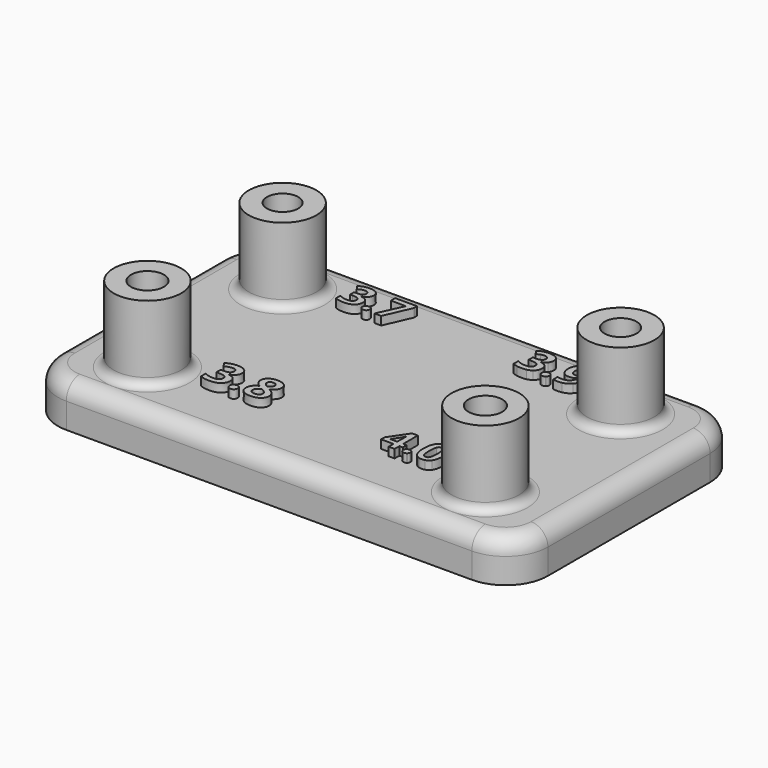
from build123d import *

# Parameters (mm, degrees)
F0_R           = 4
F0_R_2         = 1.85
F1_DEPTH       = 12
F0_R_3         = 1.95
F0_R_4         = 2
F0_R_5         = 1.9
F2_W           = 58
F2_H           = 34
F3_DEPTH       = 5
F5_R           = 5
F6_TEXT_SIZE   = 5.0406240237
F6_TEXT_SIZE_2 = 5.4685932377
F7_DEPTH       = 6
F9_R           = 2
F10_R          = 0.99999


# Not quite as in the source:
# - a fillet or chamfer is up to 0.001 mm smaller than in the source, because OpenCascade refuses the exact size
# - Text() gives the source's letters only with a copy of the font that has no kerning and outlines rounded to 1/6400 em; it was checked with that copy


with BuildPart() as f1:
    # F0 (on Top) → F1 (new body)
    with BuildSketch(Plane.XY):
        with Locations((-20, 10)):
            Circle(F0_R)
        with Locations((-20, 10)):
            Circle(F0_R_2, mode=Mode.SUBTRACT)
    extrude(amount=F1_DEPTH)


with BuildPart() as f1b:
    # F0 (on Top) → F1, piece 2 (new body)
    with BuildSketch(Plane.XY):
        with Locations((-20, -10)):
            Circle(F0_R)
        with Locations((-20, -10)):
            Circle(F0_R_3, mode=Mode.SUBTRACT)
    extrude(amount=F1_DEPTH)


with BuildPart() as f1c:
    # F0 (on Top) → F1, piece 3 (new body)
    with BuildSketch(Plane.XY):
        with Locations((20, -10)):
            Circle(F0_R)
        with Locations((20, -10)):
            Circle(F0_R_4, mode=Mode.SUBTRACT)
    extrude(amount=F1_DEPTH)


with BuildPart() as f1d:
    # F0 (on Top) → F1, piece 4 (new body)
    with BuildSketch(Plane.XY):
        with Locations((20, 10)):
            Circle(F0_R)
        with Locations((20, 10)):
            Circle(F0_R_5, mode=Mode.SUBTRACT)
    extrude(amount=F1_DEPTH)


with BuildPart() as f3:
    # F2 (on Top) → F3 (new body)
    with BuildSketch(Plane.XY):
        Rectangle(F2_W, F2_H)
    extrude(amount=F3_DEPTH)

    # F5
    f5_edges = [f3.edges().sort_by_distance(p)[0] for p in [
        (29, -17, 2.5),
        (-29, -17, 2.5),
        (-29, 17, 2.5),
        (29, 17, 2.5),
    ]]
    fillet(f5_edges, radius=F5_R)

    # F6 (on Top) → F7 (join)
    with BuildSketch(Plane.XY):
        with BuildLine():
            add(Edge.make_bspline(
                [(8.8647170825, 10), (8.6159599899, 9.9472579578), (8.308504951, 9.9472579578)],
                knots=[0.5859606644, 0.5859606644, 0.5859606644, 1, 1, 1], degree=2))
            Line((8.8647170825, 10), (7.7154605589, 10))
            add(Edge.make_bspline(
                [(8.308504951, 9.9472579578), (7.9939394248, 9.9472579578), (7.7154605589, 10)],
                knots=[0, 0, 0, 0.5050353738, 0.5050353738, 0.5050353738], degree=2))
        make_face()
        with BuildLine():
            Line((7.7154605589, 10), (8.8647170825, 10))
            add(Edge.make_bspline(
                [(9.4512491981, 10.2549198705), (9.2167654477, 10.0746420917), (8.8647170825, 10)],
                knots=[0, 0, 0, 0.5859606644, 0.5859606644, 0.5859606644], degree=2))
            add(Edge.make_bspline(
                [(9.8514189783, 11.1142802878), (9.8514189783, 10.5625817832), (9.4512491981, 10.2549198705)],
                knots=[0, 0, 0, 1, 1, 1], degree=2))
            add(Edge.make_bspline(
                [(9.6136612009, 11.7174650717), (9.8514189783, 11.4935206862), (9.8514189783, 11.1142802878)],
                knots=[0, 0, 0, 1, 1, 1], degree=2))
            add(Edge.make_bspline(
                [(8.9121083225, 11.9991745509), (9.3759034235, 11.9414094571), (9.6136612009, 11.7174650717)],
                knots=[0, 0, 0, 1, 1, 1], degree=2))
            Line((8.9121083225, 11.9991745509), (8.9121083225, 12.0142437058))
            add(Edge.make_bspline(
                [(9.5219905086, 12.3599970933), (9.3047435254, 12.1088445116), (8.9121083225, 12.0142437058)],
                knots=[0, 0, 0, 1, 1, 1], degree=2))
            add(Edge.make_bspline(
                [(9.7392374918, 12.9694606918), (9.7392374918, 12.6111496751), (9.5219905086, 12.3599970933)],
                knots=[0, 0, 0, 1, 1, 1], degree=2))
            add(Edge.make_bspline(
                [(9.3951584548, 13.6387823222), (9.7392374918, 13.3980944313), (9.7392374918, 12.9694606918)],
                knots=[0, 0, 0, 1, 1, 1], degree=2))
            add(Edge.make_bspline(
                [(8.4575221495, 13.879470213), (9.0510794178, 13.879470213), (9.3951584548, 13.6387823222)],
                knots=[0, 0, 0, 1, 1, 1], degree=2))
            add(Edge.make_bspline(
                [(7.2092938181, 13.5027413404), (7.7325283635, 13.879470213), (8.4575221495, 13.879470213)],
                knots=[0, 0, 0, 1, 1, 1], degree=2))
            Line((7.2092938181, 13.5027413404), (7.583511165, 12.9460197841))
            add(Edge.make_bspline(
                [(8.0163307809, 13.1628481797), (7.8212689424, 13.1000600343), (7.583511165, 12.9460197841)],
                knots=[0, 0, 0, 1, 1, 1], degree=2))
            add(Edge.make_bspline(
                [(8.3997570557, 13.2256363252), (8.2113926194, 13.2256363252), (8.0163307809, 13.1628481797)],
                knots=[0, 0, 0, 1, 1, 1], degree=2))
            add(Edge.make_bspline(
                [(8.9439209829, 12.7911423587), (8.9439209829, 13.2256363252), (8.3997570557, 13.2256363252)],
                knots=[0, 0, 0, 1, 1, 1], degree=2))
            add(Edge.make_bspline(
                [(8.7383944535, 12.392646929), (8.9439209829, 12.5090142919), (8.9439209829, 12.7911423587)],
                knots=[0, 0, 0, 1, 1, 1], degree=2))
            add(Edge.make_bspline(
                [(8.0883278543, 12.2762795661), (8.5328679241, 12.2762795661), (8.7383944535, 12.392646929)],
                knots=[0, 0, 0, 1, 1, 1], degree=2))
            Line((8.0883278543, 12.2762795661), (7.7928049831, 12.2762795661))
            Line((7.7928049831, 12.2762795661), (7.7928049831, 11.6559326891))
            Line((7.7928049831, 11.6559326891), (8.0833048027, 11.6559326891))
            add(Edge.make_bspline(
                [(8.7844390935, 11.543332615), (8.5646805844, 11.6559326891), (8.0833048027, 11.6559326891)],
                knots=[0, 0, 0, 1, 1, 1], degree=2))
            add(Edge.make_bspline(
                [(9.0041976025, 11.1619992783), (9.0041976025, 11.4307325408), (8.7844390935, 11.543332615)],
                knots=[0, 0, 0, 1, 1, 1], degree=2))
            add(Edge.make_bspline(
                [(8.8133216404, 10.7245751984), (9.0041976025, 10.8606161802), (9.0041976025, 11.1619992783)],
                knots=[0, 0, 0, 1, 1, 1], degree=2))
            add(Edge.make_bspline(
                [(8.2214387227, 10.5885342166), (8.6224456782, 10.5885342166), (8.8133216404, 10.7245751984)],
                knots=[0, 0, 0, 1, 1, 1], degree=2))
            add(Edge.make_bspline(
                [(7.6931811257, 10.6592755271), (7.9602400376, 10.5885342166), (8.2214387227, 10.5885342166)],
                knots=[0, 0, 0, 1, 1, 1], degree=2))
            add(Edge.make_bspline(
                [(7.2042707665, 10.8421983242), (7.4261222137, 10.7300168377), (7.6931811257, 10.6592755271)],
                knots=[0, 0, 0, 1, 1, 1], degree=2))
            Line((7.2042707665, 10.8421983242), (7.2042707665, 10.1540402502))
            add(Edge.make_bspline(
                [(7.7154605589, 10), (7.4425347504, 10.0516903301), (7.2042707665, 10.1540402502)],
                knots=[0.5050353738, 0.5050353738, 0.5050353738, 1, 1, 1], degree=2))
        make_face()
        with BuildLine():
            add(Edge.make_bspline(
                [(11.0990122142, 10), (10.9898897297, 9.9296772771), (10.8250538203, 9.9296772771)],
                knots=[0.2308775808, 0.2308775808, 0.2308775808, 1, 1, 1], degree=2))
            Line((11.0990122142, 10), (10.5431894654, 10))
            add(Edge.make_bspline(
                [(10.8250538203, 9.9296772771), (10.6538929904, 9.9296772771), (10.5431894654, 10)],
                knots=[0, 0, 0, 0.7773779948, 0.7773779948, 0.7773779948], degree=2))
        make_face()
        with BuildLine():
            Line((10.5431894654, 10), (11.0990122142, 10))
            add(Edge.make_bspline(
                [(11.1595053417, 10.0485561658), (11.131768944, 10.0211096956), (11.0990122142, 10)],
                knots=[0, 0, 0, 0.2308775808, 0.2308775808, 0.2308775808], degree=2))
            add(Edge.make_bspline(
                [(11.2796399933, 10.3742173468), (11.2796399933, 10.1674350545), (11.1595053417, 10.0485561658)],
                knots=[0, 0, 0, 1, 1, 1], degree=2))
            add(Edge.make_bspline(
                [(11.1607611046, 10.7036458166), (11.2796399933, 10.5885342166), (11.2796399933, 10.3742173468)],
                knots=[0, 0, 0, 1, 1, 1], degree=2))
            add(Edge.make_bspline(
                [(10.8250538203, 10.8187574166), (11.0418822159, 10.8187574166), (11.1607611046, 10.7036458166)],
                knots=[0, 0, 0, 1, 1, 1], degree=2))
            add(Edge.make_bspline(
                [(10.4822305462, 10.7061573424), (10.599853672, 10.8187574166), (10.8250538203, 10.8187574166)],
                knots=[0, 0, 0, 1, 1, 1], degree=2))
            add(Edge.make_bspline(
                [(10.3646074204, 10.3742173468), (10.3646074204, 10.5935572682), (10.4822305462, 10.7061573424)],
                knots=[0, 0, 0, 1, 1, 1], degree=2))
            add(Edge.make_bspline(
                [(10.484742072, 10.04604464), (10.3646074204, 10.1624120029), (10.3646074204, 10.3742173468)],
                knots=[0, 0, 0, 1, 1, 1], degree=2))
            add(Edge.make_bspline(
                [(10.5431894654, 10), (10.5114866891, 10.0201387043), (10.484742072, 10.04604464)],
                knots=[0.7773779948, 0.7773779948, 0.7773779948, 1, 1, 1], degree=2))
        make_face()
        with BuildLine():
            add(Edge.make_bspline(
                [(13.0887324097, 10), (12.838141706, 9.9472579578), (12.5412631291, 9.9472579578)],
                knots=[0.6924376574, 0.6924376574, 0.6924376574, 1, 1, 1], degree=2))
            Line((13.0887324097, 10), (12.0255631612, 10))
            Line((12.0255631612, 10), (12.0255631612, 9.9840936698))
            add(Edge.make_bspline(
                [(12.5412631291, 9.9472579578), (12.2005327931, 9.9472579578), (12.0255631612, 9.9840936698)],
                knots=[0, 0, 0, 1, 1, 1], degree=2))
        make_face()
        with BuildLine():
            Line((12.0255631612, 10), (13.0887324097, 10))
            add(Edge.make_bspline(
                [(13.9824603608, 10.5048166894), (13.6529056381, 10.1187420274), (13.0887324097, 10)],
                knots=[0, 0, 0, 0.6924376574, 0.6924376574, 0.6924376574], degree=2))
            add(Edge.make_bspline(
                [(14.4583945032, 12.1925620388), (14.4583945032, 11.0623754209), (13.9824603608, 10.5048166894)],
                knots=[0, 0, 0, 1, 1, 1], degree=2))
            add(Edge.make_bspline(
                [(14.2884479229, 13.0937812197), (14.4583945032, 12.7157965842), (14.4583945032, 12.1925620388)],
                knots=[0, 0, 0, 1, 1, 1], degree=2))
            add(Edge.make_bspline(
                [(13.8007933266, 13.6705949825), (14.1185013426, 13.4717658553), (14.2884479229, 13.0937812197)],
                knots=[0, 0, 0, 1, 1, 1], degree=2))
            add(Edge.make_bspline(
                [(13.0586374475, 13.8694241098), (13.4830853107, 13.8694241098), (13.8007933266, 13.6705949825)],
                knots=[0, 0, 0, 1, 1, 1], degree=2))
            add(Edge.make_bspline(
                [(12.1080249255, 13.512368856), (12.4575456018, 13.8694241098), (13.0586374475, 13.8694241098)],
                knots=[0, 0, 0, 1, 1, 1], degree=2))
            add(Edge.make_bspline(
                [(11.7585042492, 12.5399897769), (11.7585042492, 13.1553136023), (12.1080249255, 13.512368856)],
                knots=[0, 0, 0, 1, 1, 1], degree=2))
            add(Edge.make_bspline(
                [(12.046492543, 11.6496538746), (11.7585042492, 11.9698734163), (11.7585042492, 12.5399897769)],
                knots=[0, 0, 0, 1, 1, 1], degree=2))
            add(Edge.make_bspline(
                [(12.8342744745, 11.3294343328), (12.3344808368, 11.3294343328), (12.046492543, 11.6496538746)],
                knots=[0, 0, 0, 1, 1, 1], degree=2))
            add(Edge.make_bspline(
                [(13.3311379987, 11.4286396026), (13.1323088715, 11.3294343328), (12.8342744745, 11.3294343328)],
                knots=[0, 0, 0, 1, 1, 1], degree=2))
            add(Edge.make_bspline(
                [(13.6814958503, 11.7739744026), (13.529967126, 11.5278448724), (13.3311379987, 11.4286396026)],
                knots=[0, 0, 0, 1, 1, 1], degree=2))
            Line((13.6814958503, 11.7739744026), (13.7133085107, 11.7739744026))
            add(Edge.make_bspline(
                [(13.5534080336, 11.0711657612), (13.6923791288, 11.3260856317), (13.7133085107, 11.7739744026)],
                knots=[0, 0, 0, 1, 1, 1], degree=2))
            add(Edge.make_bspline(
                [(13.1528196657, 10.697367002), (13.4144369384, 10.8162458907), (13.5534080336, 11.0711657612)],
                knots=[0, 0, 0, 1, 1, 1], degree=2))
            add(Edge.make_bspline(
                [(12.4860095611, 10.5784881133), (12.891202393, 10.5784881133), (13.1528196657, 10.697367002)],
                knots=[0, 0, 0, 1, 1, 1], degree=2))
            add(Edge.make_bspline(
                [(12.0255631612, 10.6329045061), (12.2457402579, 10.5784881133), (12.4860095611, 10.5784881133)],
                knots=[0, 0, 0, 1, 1, 1], degree=2))
            Line((12.0255631612, 10.6329045061), (12.0255631612, 10))
        make_face()
        with BuildLine():
            add(Edge.make_bspline(
                [(13.0745437777, 13.2206132735), (12.8233911959, 13.2206132735), (12.6823271625, 13.0477365798)],
                knots=[0, 0, 0, 1, 1, 1], degree=2))
            add(Edge.make_bspline(
                [(13.4918756511, 13.0058778161), (13.3282078853, 13.2206132735), (13.0745437777, 13.2206132735)],
                knots=[0, 0, 0, 1, 1, 1], degree=2))
            add(Edge.make_bspline(
                [(13.6555434169, 12.4805503326), (13.6555434169, 12.7911423587), (13.4918756511, 13.0058778161)],
                knots=[0, 0, 0, 1, 1, 1], degree=2))
            add(Edge.make_bspline(
                [(13.4801551973, 12.1101002745), (13.6555434169, 12.2712565145), (13.6555434169, 12.4805503326)],
                knots=[0, 0, 0, 1, 1, 1], degree=2))
            add(Edge.make_bspline(
                [(13.0586374475, 11.9489440345), (13.3047669777, 11.9489440345), (13.4801551973, 12.1101002745)],
                knots=[0, 0, 0, 1, 1, 1], degree=2))
            add(Edge.make_bspline(
                [(12.6693509458, 12.1113560374), (12.7974387625, 11.9489440345), (13.0586374475, 11.9489440345)],
                knots=[0, 0, 0, 1, 1, 1], degree=2))
            add(Edge.make_bspline(
                [(12.5412631291, 12.5508730555), (12.5412631291, 12.2737680403), (12.6693509458, 12.1113560374)],
                knots=[0, 0, 0, 1, 1, 1], degree=2))
            add(Edge.make_bspline(
                [(12.6823271625, 13.0477365798), (12.5412631291, 12.874859886), (12.5412631291, 12.5508730555)],
                knots=[0, 0, 0, 1, 1, 1], degree=2))
        make_face(mode=Mode.SUBTRACT)
        Polygon((8.5467911569, -10), (9.2559562138, -10), (9.2559562138, -9.2885812406), (9.6691350075, -9.2885812406), (9.6691350075, -8.7251556128), (9.2559562138, -8.7251556128), (9.2559562138, -6.5676110753), (8.5873578021, -6.5676110753), (7.0818845246, -8.7837518781), (7.0818845246, -9.2885812406), (8.5467911569, -9.2885812406), align=None)
        with BuildLine():
            Line((8.5467911569, -8.1429491307), (8.5467911569, -8.7251556128))
            Line((8.5467911569, -8.7251556128), (7.7204335694, -8.7251556128))
            Line((7.7204335694, -8.7251556128), (8.3499678042, -7.774093153))
            add(Edge.make_bspline(
                [(8.5588109036, -7.3984760678), (8.4716677399, -7.5915432496), (8.3499678042, -7.774093153)],
                knots=[0, 0, 0, 1, 1, 1], degree=2))
            Line((8.5588109036, -7.3984760678), (8.5775917579, -7.3984760678))
            add(Edge.make_bspline(
                [(8.5588109036, -7.7203799099), (8.5708306504, -7.4435501181), (8.5775917579, -7.3984760678)],
                knots=[0, 0, 0, 1, 1, 1], degree=2))
            add(Edge.make_bspline(
                [(8.5467911569, -8.1429491307), (8.5467911569, -7.9972097017), (8.5588109036, -7.7203799099)],
                knots=[0, 0, 0, 1, 1, 1], degree=2))
        make_face(mode=Mode.SUBTRACT)
        with BuildLine():
            add(Edge.make_bspline(
                [(10.6782238335, -10), (10.5803034316, -10.0631036703), (10.4323889247, -10.0631036703)],
                knots=[0.2308775808, 0.2308775808, 0.2308775808, 1, 1, 1], degree=2))
            Line((10.6782238335, -10), (10.1794596496, -10))
            add(Edge.make_bspline(
                [(10.4323889247, -10.0631036703), (10.2787987885, -10.0631036703), (10.1794596496, -10)],
                knots=[0, 0, 0, 0.7773779948, 0.7773779948, 0.7773779948], degree=2))
        make_face()
        with BuildLine():
            Line((10.1794596496, -10), (10.6782238335, -10))
            add(Edge.make_bspline(
                [(10.7325069757, -9.9564284181), (10.7076178869, -9.9810573423), (10.6782238335, -10)],
                knots=[0, 0, 0, 0.2308775808, 0.2308775808, 0.2308775808], degree=2))
            add(Edge.make_bspline(
                [(10.8403090792, -9.6641983258), (10.8403090792, -9.8497531659), (10.7325069757, -9.9564284181)],
                knots=[0, 0, 0, 1, 1, 1], degree=2))
            add(Edge.make_bspline(
                [(10.733633827, -9.3685876798), (10.8403090792, -9.4718823782), (10.8403090792, -9.6641983258)],
                knots=[0, 0, 0, 1, 1, 1], degree=2))
            add(Edge.make_bspline(
                [(10.4323889247, -9.2652929813), (10.6269585748, -9.2652929813), (10.733633827, -9.3685876798)],
                knots=[0, 0, 0, 1, 1, 1], degree=2))
            add(Edge.make_bspline(
                [(10.1247585319, -9.3663339772), (10.2303069328, -9.2652929813), (10.4323889247, -9.2652929813)],
                knots=[0, 0, 0, 1, 1, 1], degree=2))
            add(Edge.make_bspline(
                [(10.0192101309, -9.6641983258), (10.0192101309, -9.4673749732), (10.1247585319, -9.3663339772)],
                knots=[0, 0, 0, 1, 1, 1], degree=2))
            add(Edge.make_bspline(
                [(10.1270122344, -9.9586821206), (10.0192101309, -9.8542605709), (10.0192101309, -9.6641983258)],
                knots=[0, 0, 0, 1, 1, 1], degree=2))
            add(Edge.make_bspline(
                [(10.1794596496, -10), (10.1510113548, -9.9819286554), (10.1270122344, -9.9586821206)],
                knots=[0.7773779948, 0.7773779948, 0.7773779948, 1, 1, 1], degree=2))
        make_face()
        with BuildLine():
            add(Edge.make_bspline(
                [(12.8570365656, -10), (12.6890842324, -10.0473277527), (12.4862631466, -10.0473277527)],
                knots=[0.6691374514, 0.6691374514, 0.6691374514, 1, 1, 1], degree=2))
            Line((12.8570365656, -10), (12.1302543992, -10))
            add(Edge.make_bspline(
                [(12.4862631466, -10.0473277527), (12.2927418034, -10.0473277527), (12.1302543992, -10)],
                knots=[0, 0, 0, 0.3256694736, 0.3256694736, 0.3256694736], degree=2))
        make_face()
        with BuildLine():
            Line((12.1302543992, -10), (12.8570365656, -10))
            add(Edge.make_bspline(
                [(13.3937540245, -9.6149924877), (13.1967038885, -9.9042842051), (12.8570365656, -10)],
                knots=[0, 0, 0, 0.6691374514, 0.6691374514, 0.6691374514], degree=2))
            add(Edge.make_bspline(
                [(13.6882378193, -8.2841811548), (13.6882378193, -9.1826572226), (13.3937540245, -9.6149924877)],
                knots=[0, 0, 0, 1, 1, 1], degree=2))
            add(Edge.make_bspline(
                [(13.3843635973, -6.9642627173), (13.6882378193, -7.4150032196), (13.6882378193, -8.2841811548)],
                knots=[0, 0, 0, 1, 1, 1], degree=2))
            add(Edge.make_bspline(
                [(12.4862631466, -6.5135222151), (13.0804893754, -6.5135222151), (13.3843635973, -6.9642627173)],
                knots=[0, 0, 0, 1, 1, 1], degree=2))
            add(Edge.make_bspline(
                [(11.5825284396, -6.9443550118), (11.8762610002, -6.5135222151), (12.4862631466, -6.5135222151)],
                knots=[0, 0, 0, 1, 1, 1], degree=2))
            add(Edge.make_bspline(
                [(11.2887958789, -8.2841811548), (11.2887958789, -7.3751878085), (11.5825284396, -6.9443550118)],
                knots=[0, 0, 0, 1, 1, 1], degree=2))
            add(Edge.make_bspline(
                [(11.5904163984, -9.6010946555), (11.2887958789, -9.1548615583), (11.2887958789, -8.2841811548)],
                knots=[0, 0, 0, 1, 1, 1], degree=2))
            add(Edge.make_bspline(
                [(12.1302543992, -10), (11.793808322, -9.9020032548), (11.5904163984, -9.6010946555)],
                knots=[0.3256694736, 0.3256694736, 0.3256694736, 1, 1, 1], degree=2))
        make_face()
        with BuildLine():
            add(Edge.make_bspline(
                [(12.0099806825, -8.2841811548), (12.0099806825, -8.9152178579), (12.1189096373, -9.1886670959)],
                knots=[0, 0, 0, 1, 1, 1], degree=2))
            add(Edge.make_bspline(
                [(12.1200364885, -7.3766902769), (12.0099806825, -7.6523932174), (12.0099806825, -8.2841811548)],
                knots=[0, 0, 0, 1, 1, 1], degree=2))
            add(Edge.make_bspline(
                [(12.4862631466, -7.1009873363), (12.2300922945, -7.1009873363), (12.1200364885, -7.3766902769)],
                knots=[0, 0, 0, 1, 1, 1], degree=2))
            add(Edge.make_bspline(
                [(12.8513629534, -7.3766902769), (12.7371753595, -7.1009873363), (12.4862631466, -7.1009873363)],
                knots=[0, 0, 0, 1, 1, 1], degree=2))
            add(Edge.make_bspline(
                [(12.9655505473, -8.2841811548), (12.9655505473, -7.6523932174), (12.8513629534, -7.3766902769)],
                knots=[0, 0, 0, 1, 1, 1], degree=2))
            add(Edge.make_bspline(
                [(12.8528654218, -9.1852865422), (12.9655505473, -8.9084567504), (12.9655505473, -8.2841811548)],
                knots=[0, 0, 0, 1, 1, 1], degree=2))
            add(Edge.make_bspline(
                [(12.4862631466, -9.462116334), (12.7401802962, -9.462116334), (12.8528654218, -9.1852865422)],
                knots=[0, 0, 0, 1, 1, 1], degree=2))
            add(Edge.make_bspline(
                [(12.1189096373, -9.1886670959), (12.227838592, -9.462116334), (12.4862631466, -9.462116334)],
                knots=[0, 0, 0, 1, 1, 1], degree=2))
        make_face(mode=Mode.SUBTRACT)
        with Locations((-14, 10)):
            Text('3.7', F6_TEXT_SIZE, font='Open Sans', font_style=FontStyle.BOLD, text_align=(TextAlign.LEFT, TextAlign.BOTTOM))
        with Locations((-14, -10)):
            Text('3.8', F6_TEXT_SIZE_2, font='Open Sans', font_style=FontStyle.BOLD, text_align=(TextAlign.LEFT, TextAlign.BOTTOM))
    extrude(amount=F7_DEPTH)


with BuildPart() as f1d_1:
    # F4: moved
    add(f1d.part.moved(Location((0, 0, 2))))


with BuildPart() as f1c_1:
    # F4: moved
    add(f1c.part.moved(Location((0, 0, 2))))


with BuildPart() as f1b_1:
    # F4: moved
    add(f1b.part.moved(Location((0, 0, 2))))


with BuildPart() as f1_1:
    # F4: moved
    add(f1.part.moved(Location((0, 0, 2))))

    # F8: union F1b, F1c, F1d, F3
    add(f1b_1.part)
    add(f1c_1.part)
    add(f1d_1.part)
    add(f3.part)

    # F9
    f9_edges = [f1_1.edges().sort_by_distance(p)[0] for p in [
        (0, -17, 5),
    ]]
    fillet(f9_edges, radius=F9_R)

    # F10 (radius 1 in the source; OpenCascade refuses exactly that, so slightly less here)
    f10_edges = [f1_1.edges().sort_by_distance(p)[0] for p in [
        (-24, -10, 5),
        (-24, 10, 5),
        (16, -10, 5),
        (16, 10, 5),
    ]]
    fillet(f10_edges, radius=F10_R)


solid = f1_1.part
